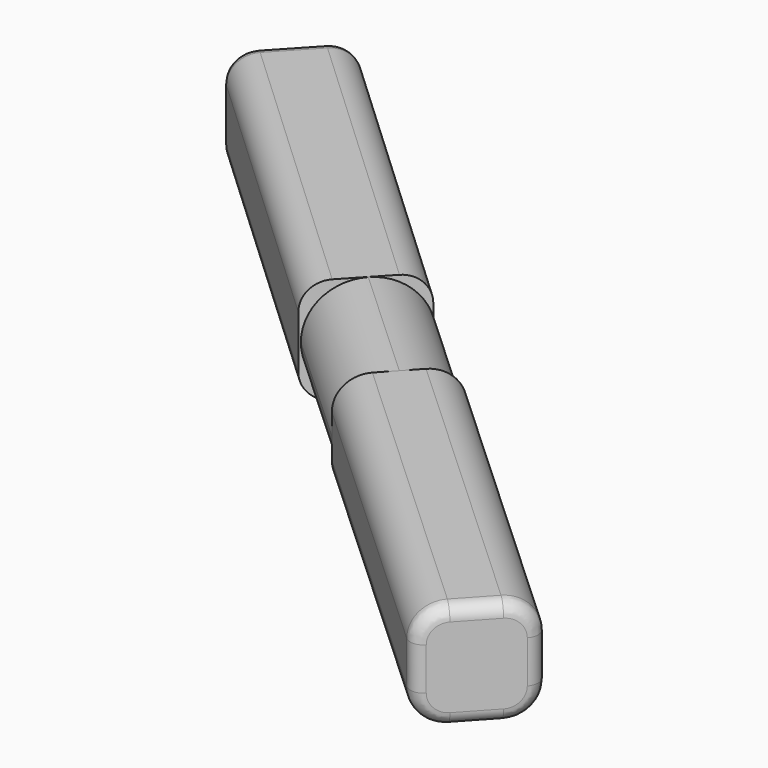
from build123d import *

# Parameters (mm, degrees)
F1_DEPTH = 3.9878
F3_DEPTH = 5.9944
F4_R     = 1.2
F5_R     = 1
F6_R     = 0.5
F6_2_R   = 0.5


with BuildPart() as f1:
    # F0 (on Top) → F1 (new body)
    with BuildSketch(Plane.XY):
        Polygon((11.0322314148, -10.163162402), (0, 0), (-2.7019106018, -2.9329554957), (8.330320813, -13.0961178978), align=None)
    extrude(amount=F1_DEPTH)

    # F2 (on face) → F3 (join)
    with BuildSketch(Plane(origin=(0, 0, 0), x_dir=(-0.6775441601, -0.7354820943, 0), z_dir=(-0.7354820943, 0.6775441601, 0))):
        Polygon((3.9878, 1.9939), (1.9939, 3.9878), (1.9939, 1.9939), align=None)
        with BuildLine():
            ThreePointArc((3.9878, 1.9939), (3.403800211, 3.403800211), (1.9939, 3.9878))
            Line((1.9939, 3.9878), (3.9878, 1.9939))
        make_face()
        with BuildLine():
            Line((1.9939, 1.9939), (1.9939, 3.9878))
            ThreePointArc((1.9939, 3.9878), (0.583999789, 3.403800211), (0, 1.9939))
            Line((0, 1.9939), (1.9939, 1.9939))
        make_face()
        with BuildLine():
            Line((3.9878, 1.9939), (1.9939, 1.9939))
            Line((1.9939, 1.9939), (1.9939, 0))
            ThreePointArc((1.9939, 0), (3.403800211, 0.583999789), (3.9878, 1.9939))
        make_face()
        Polygon((1.9939, 0), (1.9939, 1.9939), (0, 1.9939), align=None)
        with BuildLine():
            Line((1.9939, 0), (0, 1.9939))
            ThreePointArc((0, 1.9939), (0.583999789, 0.583999789), (1.9939, 0))
        make_face()
    extrude(amount=F3_DEPTH)

    # F4
    f4_edges = [f1.edges().sort_by_distance(p)[0] for p in [
        (5.516116, -5.081581, 3.9878),
        (5.516116, -5.081581, 0),
        (2.814205, -8.014537, 3.9878),
        (2.814205, -8.014537, 0),
    ]]
    fillet(f4_edges, radius=F4_R)

    # F6
    f6_edges = [f1.edges().sort_by_distance(p)[0] for p in [
        (8.330321, -13.096118, 1.9939),
        (8.568459, -12.837617, 0.351472),
        (8.568459, -12.837617, 3.636328),
        (9.681276, -11.62964, 0),
        (9.681276, -11.62964, 3.9878),
        (10.794094, -10.421664, 0.351472),
        (10.794094, -10.421664, 3.636328),
        (11.032231, -10.163162, 1.9939),
    ]]
    fillet(f6_edges, radius=F6_R)


with BuildPart() as f1b:
    # F0 (on Top) → F1, piece 2 (new body)
    with BuildSketch(Plane.XY):
        Polygon((-7.1761466079, 1.0931465663), (-4.4561972482, 4.0093811798), (-15.4338702201, 14.2481714444), (-18.1538195797, 11.3319368309), align=None)
    extrude(amount=F1_DEPTH)

    # F5
    f5_edges = [f1b.edges().sort_by_distance(p)[0] for p in [
        (-12.664983, 6.212542, 3.9878),
        (-12.664983, 6.212542, 0),
        (-9.945034, 9.128776, 0),
        (-9.945034, 9.128776, 3.9878),
    ]]
    fillet(f5_edges, radius=F5_R)

    # F6#2
    f6_2_edges = [f1b.edges().sort_by_distance(p)[0] for p in [
        (-15.43387, 14.248171, 1.9939),
        (-15.633643, 14.033982, 0.292893),
        (-15.633643, 14.033982, 3.694907),
        (-16.793845, 12.790054, 0),
        (-16.793845, 12.790054, 3.9878),
        (-17.954047, 11.546126, 0.292893),
        (-17.954047, 11.546126, 3.694907),
        (-18.15382, 11.331937, 1.9939),
    ]]
    fillet(f6_2_edges, radius=F6_2_R)


solid = Compound([f1.part, f1b.part])
